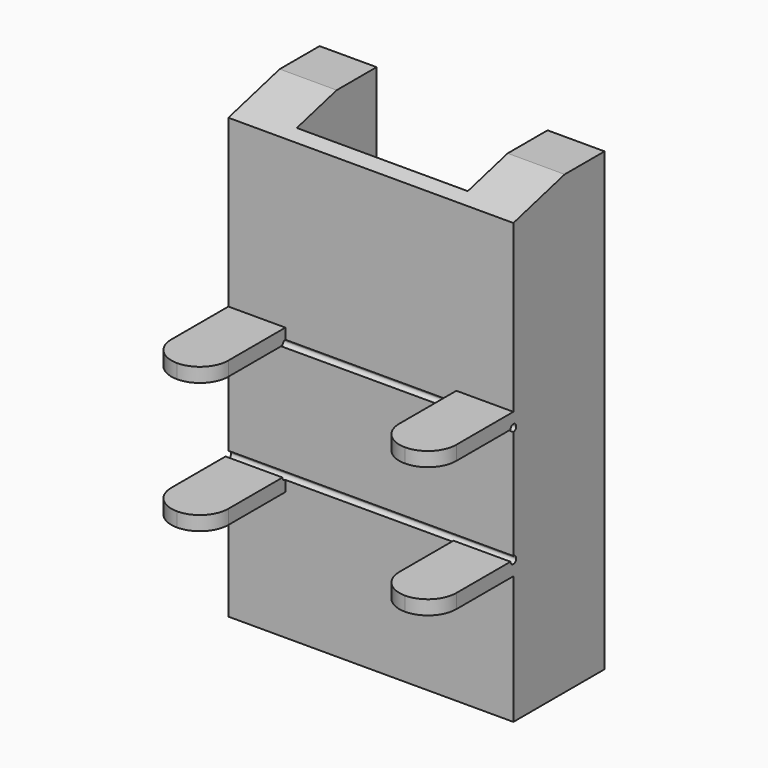
from build123d import *

# Parameters (mm, degrees)
F1_DEPTH = 203.2
F2_W     = 44.45
F2_H     = 57.15
F3_DEPTH = 127.001
F4_R     = 12.69999


# Not quite as in the source:
# - a fillet or chamfer is up to 0.001 mm smaller than in the source, because OpenCascade refuses the exact size
# - a feature of the source that left no trace in its solid (it failed there, or was rolled back) is left out


with BuildPart() as f1:
    # F0 (on Top) → F1 (new body)
    with BuildSketch(Plane.XY):
        Polygon((-38.1, 0), (0, 0), (38.1, 0), (38.1, -44.45), (63.5, -44.45), (63.5, 50.8), (38.1, 50.8), (38.1, 6.35), (0, 6.35), (-38.1, 6.35), (-38.1, 50.8), (-63.5, 50.8), (-63.5, -44.45), (-38.1, -44.45), align=None)
    extrude(amount=F1_DEPTH)

    # F2 (on face) → F3 (cut, through all)
    with BuildSketch(Plane.YZ.offset(63.5)):
        with BuildLine():
            Line((-44.45, 115.316), (-44.45, 63.5))
            Line((-44.45, 63.5), (-1.5875, 63.5))
            ThreePointArc((-1.5875, 63.5), (-1.1225320151, 64.6225320151), (0, 65.0875))
            Line((0, 65.0875), (0, 113.7285))
            ThreePointArc((0, 113.7285), (-1.1225320151, 114.1934679849), (-1.5875, 115.316))
            Line((-1.5875, 115.316), (-44.45, 115.316))
        make_face()
        with BuildLine():
            ThreePointArc((0, 65.0875), (-1.1225320151, 64.6225320151), (-1.5875, 63.5))
            Line((-1.5875, 63.5), (0, 63.5))
            Line((0, 63.5), (0, 65.0875))
        make_face()
        with Locations((-22.225, 28.575)):
            Rectangle(F2_W, F2_H)
        Polygon((-44.45, 203.2), (-44.45, 184.15), (0, 195.7456521739), (0, 203.2), align=None)
        with BuildLine():
            Line((0, 115.316), (0, 113.7285))
            ThreePointArc((0, 113.7285), (1.1225320151, 114.1934679849), (1.5875, 115.316))
            ThreePointArc((1.5875, 115.316), (1.1225320151, 116.4385320151), (0, 116.9035))
            Line((0, 116.9035), (0, 115.316))
        make_face()
        with BuildLine():
            ThreePointArc((0, 116.9035), (-1.1225320151, 116.4385320151), (-1.5875, 115.316))
            Line((-1.5875, 115.316), (0, 115.316))
            Line((0, 115.316), (0, 116.9035))
        make_face()
        with BuildLine():
            Line((0, 115.316), (-1.5875, 115.316))
            ThreePointArc((-1.5875, 115.316), (-1.1225320151, 114.1934679849), (0, 113.7285))
            Line((0, 113.7285), (0, 115.316))
        make_face()
        with BuildLine():
            Line((0, 65.0875), (0, 63.5))
            Line((0, 63.5), (0, 61.9125))
            ThreePointArc((0, 61.9125), (1.1225320151, 62.3774679849), (1.5875, 63.5))
            ThreePointArc((1.5875, 63.5), (1.1225320151, 64.6225320151), (0, 65.0875))
        make_face()
        with BuildLine():
            Line((0, 63.5), (-1.5875, 63.5))
            ThreePointArc((-1.5875, 63.5), (-1.1225320151, 62.3774679849), (0, 61.9125))
            Line((0, 61.9125), (0, 63.5))
        make_face()
        Polygon((0, 203.2), (0, 195.7456521739), (28.575, 203.2), align=None)
        Polygon((-44.45, 184.15), (-44.45, 121.666), (0, 121.666), (0, 195.7456521739), align=None)
    extrude(amount=-F3_DEPTH, mode=Mode.SUBTRACT)

    # F4 (radius 12.7 in the source; OpenCascade refuses exactly that, so slightly less here)
    f4_edges = [f1.edges().sort_by_distance(p)[0] for p in [
        (38.1, -44.45, 118.491),
        (63.5, -44.45, 118.491),
        (-63.5, -44.45, 118.491),
        (-38.1, -44.45, 118.491),
        (-38.1, -44.45, 60.325),
        (-63.5, -44.45, 60.325),
        (38.1, -44.45, 60.325),
        (63.5, -44.45, 60.325),
    ]]
    fillet(f4_edges, radius=F4_R)


solid = f1.part
